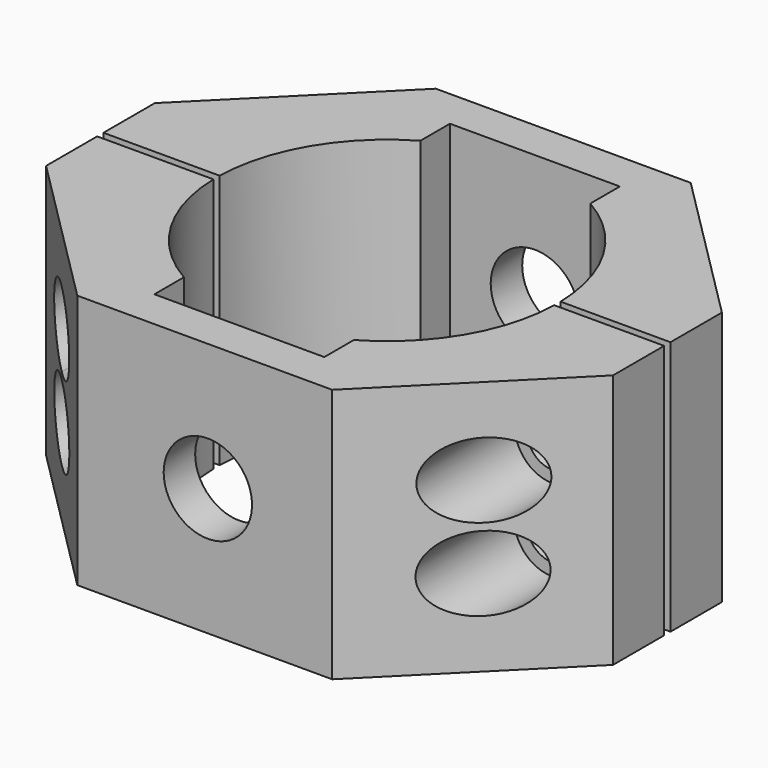
from build123d import *
from build123d import SkipClean  # not in build123d's __all__

# Parameters (mm, degrees)
F1_DEPTH  = 19.05
F3_DEPTH  = 66.9907422194
F4_R      = 5.60689081
F5_DEPTH  = 25.4
F7_DEPTH  = 25.4
F8_W      = 110.2635304305
F8_H      = 1.1740395275
F9_DEPTH  = 38.1010001
F10_W     = 25.4
F10_H     = 6.3003107457
F11_DEPTH = 38.1010001


with BuildPart() as f1:
    # F0 (on Top) → F1 (new body, symmetric)
    with BuildSketch(Plane.XY):
        Polygon((41.9069059193, 10.174138844), (18.5861736536, 33.4948711097), (0, 33.4948711097), (-19.5138263464, 33.4948711097), (-42.8505130112, 10.1581844449), (-42.8505130112, 0), (-42.8505130112, -10.1581844449), (-19.5138263464, -33.4948711097), (18.5861736536, -33.4948711097), (41.9069059193, -10.174138844), align=None)
        with BuildLine():
            ThreePointArc((25.48255, 0), (-18.0188839069, -18.0188839069), (0, 25.48255))
            ThreePointArc((0, 25.48255), (18.0188839069, 18.0188839069), (25.48255, 0))
        make_face(mode=Mode.SUBTRACT)
    extrude(amount=F1_DEPTH, both=True)

    # F2 (on face) → F3 (cut, through all)
    with BuildSketch(Plane(origin=(0, 33.4948711097, 0), x_dir=(-1, 0, 0), z_dir=(0, 1, 0))):
        with BuildLine():
            ThreePointArc((31.1872387667, 2.2823126413), (33.8813156031, 3.398235805), (34.9972387667, 6.0923126413))
            ThreePointArc((34.9972387667, 6.0923126413), (28.4931619304, 8.7863894776), (31.1872387667, 2.2823126413))
        make_face()
        with BuildLine():
            ThreePointArc((34.9972387667, -6.0923126413), (33.8813156031, -3.398235805), (31.1872387667, -2.2823126413))
            ThreePointArc((31.1872387667, -2.2823126413), (28.4931619304, -8.7863894776), (34.9972387667, -6.0923126413))
        make_face()
        with BuildLine():
            ThreePointArc((-27.3772387667, -6.0923126413), (-28.4931619304, -3.398235805), (-31.1872387667, -2.2823126413))
            ThreePointArc((-31.1872387667, -2.2823126413), (-33.8813156031, -8.7863894776), (-27.3772387667, -6.0923126413))
        make_face()
        with BuildLine():
            ThreePointArc((-27.3772387667, 6.0923126413), (-33.8813156031, 8.7863894776), (-31.1872387667, 2.2823126413))
            ThreePointArc((-31.1872387667, 2.2823126413), (-28.4931619304, 3.398235805), (-27.3772387667, 6.0923126413))
        make_face()
        with BuildLine():
            ThreePointArc((-6.6042914247, 0), (0, -6.6042914247), (6.6042914247, 0))
            Line((6.6042914247, 0), (-6.6042914247, 0))
        make_face()
        with BuildLine():
            Line((-6.6042914247, 0), (6.6042914247, 0))
            ThreePointArc((6.6042914247, 0), (0, 6.6042914247), (-6.6042914247, 0))
        make_face()
    extrude(amount=-F3_DEPTH, mode=Mode.SUBTRACT)

    # F4 (on face) → F5 (cut)
    with BuildSketch(Plane.XZ.offset(33.4948711097)):
        with BuildLine():
            ThreePointArc((-31.1506315094, 0.5265610691), (-27.2071362658, 2.1802747004), (-25.5764710601, 6.1333563462))
            ThreePointArc((-25.5764710601, 6.1333563462), (-35.1595874746, 10.086437992), (-31.1506315094, 0.5265610691))
        make_face()
        with BuildLine():
            ThreePointArc((-25.5048626079, -6.1333563462), (-27.1586717722, -2.1571307417), (-31.1444837787, -0.5265610691))
            ThreePointArc((-31.1444837787, -0.5265610691), (-35.0648350638, -10.1095819506), (-25.5048626079, -6.1333563462))
        make_face()
        with Locations((31.111753418, -6.1333563462)):
            Circle(F4_R)
        with Locations((31.1833618702, 6.1333563462)):
            Circle(F4_R)
    extrude(amount=-F5_DEPTH, mode=Mode.SUBTRACT)

    # F6 (on face) → F7 (cut)
    with BuildSketch(Plane(origin=(0, 33.4948711097, 0), x_dir=(-1, 0, 0), z_dir=(0, 1, 0))):
        with BuildLine():
            ThreePointArc((-31.2060154974, 0.3319311278), (-27.2413449843, 1.9741514247), (-25.5991246874, 5.9388219379))
            ThreePointArc((-25.5991246874, 5.9388219379), (-35.1706860106, 9.903492451), (-31.2060154974, 0.3319311278))
        make_face()
        with BuildLine():
            ThreePointArc((36.8129063075, 5.9388219379), (27.2413449843, 9.903492451), (31.2060154974, 0.3319311278))
            ThreePointArc((31.2060154974, 0.3319311278), (35.1706860106, 1.9741514247), (36.8129063075, 5.9388219379))
        make_face()
        with BuildLine():
            ThreePointArc((36.8129063075, -6.118518766), (35.1706860106, -2.1538482529), (31.2060154974, -0.511627956))
            ThreePointArc((31.2060154974, -0.511627956), (27.2413449843, -10.0831892792), (36.8129063075, -6.118518766))
        make_face()
        with BuildLine():
            ThreePointArc((-25.5991246874, -6.118518766), (-27.2413449843, -2.1538482529), (-31.2060154974, -0.511627956))
            ThreePointArc((-31.2060154974, -0.511627956), (-35.1706860106, -10.0831892792), (-25.5991246874, -6.118518766))
        make_face()
    extrude(amount=-F7_DEPTH, mode=Mode.SUBTRACT)

    # F8 (on face) → F9 (cut, through all)
    with BuildSketch(Plane(origin=(0, 0, -19.05), x_dir=(1, 0, 0), z_dir=(0, 0, -1))):
        with Locations((5.5118532782, 0.0261101668)):
            Rectangle(F8_W, F8_H)
    extrude(amount=-F9_DEPTH, mode=Mode.SUBTRACT)

    # F10 (on face) → F11 (cut, through all)
    with BuildSketch(Plane.XY.offset(19.05)):
        Polygon((0, -21.3100345684), (-12.7, -21.3100345684), (-12.7, -27.6103453141), (12.7, -27.6103453141), (12.7, -21.3100345684), align=None)
        with Locations((0, 24.4601899413)):
            Rectangle(F10_W, F10_H)
    with SkipClean():  # cleaning this boolean's faces spoils the solid; the shape is the same uncleaned
        extrude(amount=-F11_DEPTH, mode=Mode.SUBTRACT)


solid = f1.part
